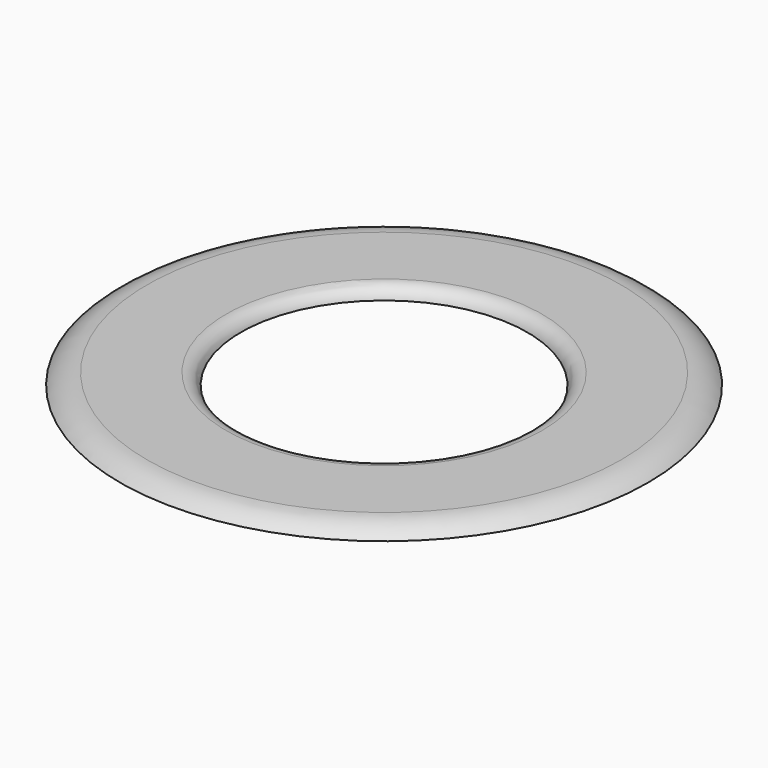
from build123d import *

# Parameters (mm, degrees)
F0_R     = 35
F0_R_2   = 19
F1_DEPTH = 1.5


# Not quite as in the source:
# - a fillet or chamfer that OpenCascade refuses, or shapes differently, is made with other operations: its cross-section is extruded or revolved along the edge and cut away or added


with BuildPart() as f1:
    # F0 (on Top) → F1 (new body)
    with BuildSketch(Plane.XY):
        Circle(F0_R)
        Circle(F0_R_2, mode=Mode.SUBTRACT)
    extrude(amount=F1_DEPTH)

    # F2: fillet of radius 2 on 1 edges, made by hand

    # F2_s1 → F2_t2 (revolve, cut)
    with BuildSketch(Plane.XZ):
        with BuildLine():
            ThreePointArc((19, 0), (19.7117468017, 1.0811388301), (20.9364916731, 1.5))
            Line((20.9364916731, 1.5), (19, 1.5))
            Line((19, 1.5), (19, 0))
        make_face()
    revolve(axis=Axis((0, 0, 1.5), (0, 0, 1)), mode=Mode.SUBTRACT)

    # F3: fillet of radius 5 on 1 edges, made by hand

    # F3_s1 → F3_t2 (revolve, cut)
    with BuildSketch(Plane.XZ):
        with BuildLine():
            ThreePointArc((35, 0), (33.3657774588, 1.1097722286), (31.4292857857, 1.5))
            Line((31.4292857857, 1.5), (35, 1.5))
            Line((35, 1.5), (35, 0))
        make_face()
    revolve(axis=Axis((0, 0, 1.5), (0, 0, 1)), mode=Mode.SUBTRACT)


solid = f1.part
